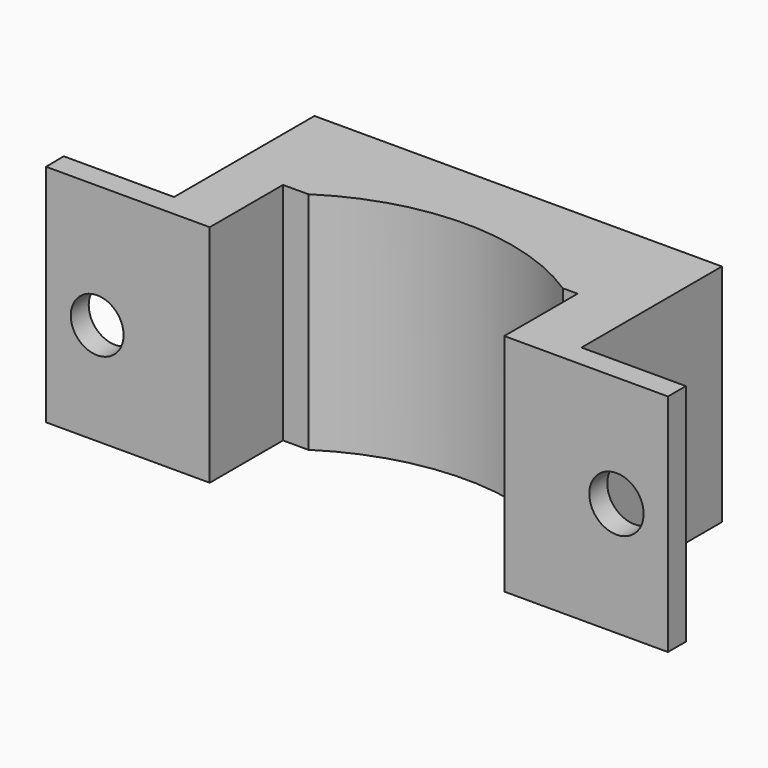
from build123d import *

# Parameters (mm, degrees)
F1_DEPTH = 17.4625
F2_R     = 2.1078217737
F3_DEPTH = 25.4
F4_R     = 2.0502205364
F5_DEPTH = 25.4
F7_DEPTH = 25.4


# Not quite as in the source:
# - a length typed as a fraction of an inch, garbled in the dataset ("3 / 203.2 mm" for 3/8 in), is restored
# - a feature names something its author has since deleted; it is built from what else it names


with BuildPart() as f1:
    # F0 (on Top) → F1 (new body)
    with BuildSketch(Plane.XY):
        Polygon((-14.4545807227, 0), (-1.7545807227, 0), (-1.7545807227, 1.7429942964), (-9.8568759859, 1.7429942964), (-9.8568759859, 15.3656043112), (-41.4793491364, 15.3656043112), (-41.4793491364, 1.7429942964), (-50.0414928719, 1.7429942964), (-50.0145807227, 0), (-37.3145807227, 0), (-37.3145807227, 7.112), (-14.4545807227, 7.112), align=None)
    extrude(amount=F1_DEPTH)

    # F2 (on face) → F3 (cut)
    with BuildSketch(Plane(origin=(0, 1.7429942964, 0), x_dir=(-1, 0, 0), z_dir=(0, 1, 0))):
        with Locations((5.7487357408, 8.8277282193)):
            Circle(F2_R)
    extrude(amount=-F3_DEPTH, mode=Mode.SUBTRACT)

    # F4 (on face) → F5 (cut)
    with BuildSketch(Plane(origin=(0, 1.7429942964, 0), x_dir=(-1, 0, 0), z_dir=(0, 1, 0))):
        with Locations((46.049553901, 7.9207858071)):
            Circle(F4_R)
    extrude(amount=-F5_DEPTH, mode=Mode.SUBTRACT)

    # F6 (on face) → F7 (cut)
    with BuildSketch(Plane(origin=(0, 0, 0), x_dir=(1, 0, 0), z_dir=(0, 0, -1))):
        with BuildLine():
            Line((-15.6063264408, -7.112), (-35.3541379623, -7.112))
            ThreePointArc((-35.3541379623, -7.112), (-25.4802322015, -10.0417717978), (-15.6063264408, -7.112))
        make_face()
    extrude(amount=-F7_DEPTH, mode=Mode.SUBTRACT)


solid = f1.part
